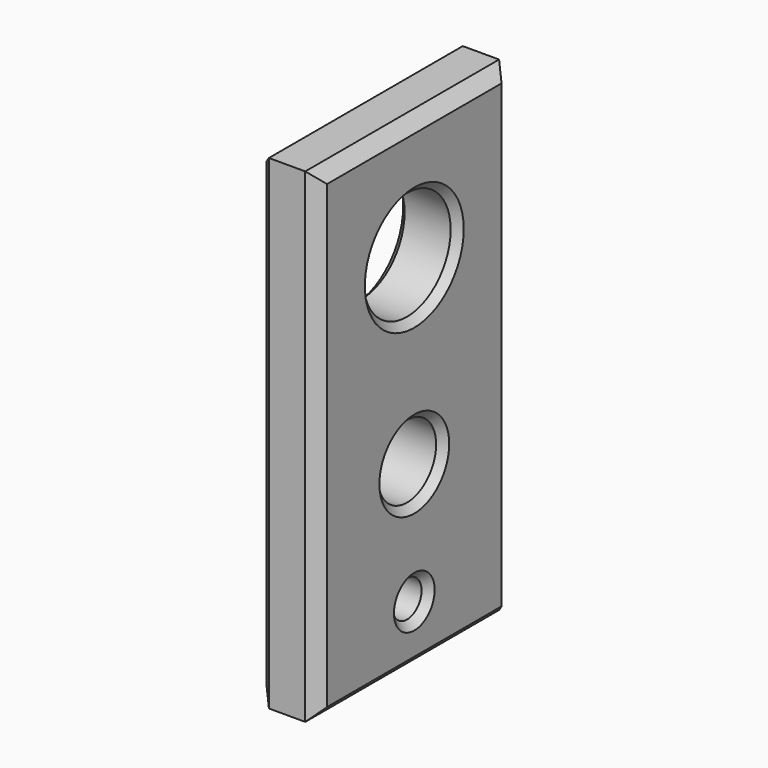
from build123d import *

# Parameters (mm, degrees)
F0_W     = 100
F0_H     = 200
F0_R     = 7.5
F0_R_2   = 15
F0_R_3   = 22.5
F1_DEPTH = 25
F2_SIZE  = 5
F3_DEPTH = 25
F4_SIZE  = 5
F5_SIZE  = 3


# Not quite as in the source:
# - a feature names something its author has since deleted; it is built from what else it names


with BuildPart() as f1:
    # F0 (on Right) → F1 (new body)
    with BuildSketch(Plane.YZ):
        Rectangle(F0_W, F0_H)
        with Locations((0, -75)):
            Circle(F0_R, mode=Mode.SUBTRACT)
        with Locations((0, -25)):
            Circle(F0_R_2, mode=Mode.SUBTRACT)
        with Locations((0, 50)):
            Circle(F0_R_3, mode=Mode.SUBTRACT)
    extrude(amount=F1_DEPTH)

    # F2
    f2_edges = [f1.edges().sort_by_distance(p)[0] for p in [
        (25, 50, 0),
        (0, 50, 0),
        (12.5, 22.5, 50),
        (0, -22.5, 50),
        (25, -22.5, 50),
        (12.5, 7.5, -75),
        (0, -7.5, -75),
        (25, -7.5, -75),
        (0, -50, 0),
        (25, -50, 0),
        (25, 0, -100),
        (0, 0, -100),
        (0, 0, 100),
        (25, 0, 100),
    ]]
    chamfer(f2_edges, length=F2_SIZE)

    # F0 (on Right) → F3 (join)
    with BuildSketch(Plane.YZ):
        Rectangle(F0_W, F0_H)
        with Locations((0, -75)):
            Circle(F0_R, mode=Mode.SUBTRACT)
        with Locations((0, -25)):
            Circle(F0_R_2, mode=Mode.SUBTRACT)
        with Locations((0, 50)):
            Circle(F0_R_3, mode=Mode.SUBTRACT)
    extrude(amount=F3_DEPTH)

    # F4
    f4_edges = [f1.edges().sort_by_distance(p)[0] for p in [
        (25, 0, 100),
        (25, -50, 0),
        (25, 0, -100),
        (25, 50, 0),
        (0, -50, 0),
        (0, 0, 100),
        (0, 50, 0),
        (0, 0, -100),
    ]]
    chamfer(f4_edges, length=F4_SIZE)

    # F5
    f5_edges = [f1.edges().sort_by_distance(p)[0] for p in [
        (0, -22.5, 50),
        (12.5, 22.5, 50),
        (25, -22.5, 50),
        (12.5, 15, -25),
        (0, -15, -25),
        (25, -15, -25),
        (0, -7.5, -75),
        (12.5, 7.5, -75),
        (25, -7.5, -75),
    ]]
    chamfer(f5_edges, length=F5_SIZE)


solid = f1.part
